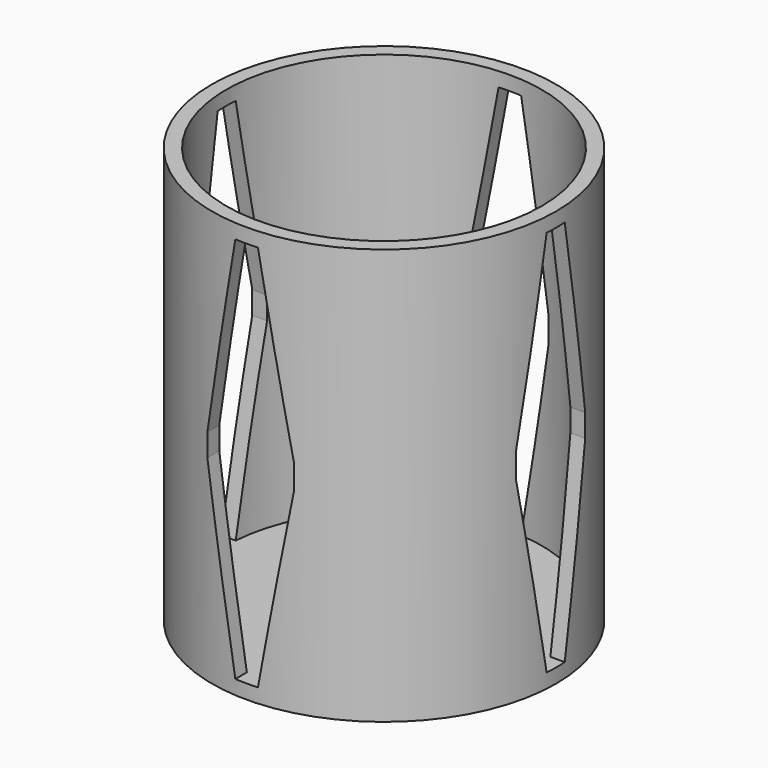
from build123d import *

# Parameters (mm, degrees)
F0_R            = 38.1
F1_DEPTH        = 3.175
F2_R            = 38.1
F2_R_2          = 34.925
F3_DEPTH        = 88.9
F5_DEPTH        = 38.101
F5_COPIES_COUNT = 4


# Not quite as in the source:
# - a pattern or mirror of a feature is missing from the dataset's text; its kind, count and spacing are read off the source's solid


with BuildPart() as f1:
    # F0 (on Top) → F1 (new body)
    with BuildSketch(Plane.XY):
        Circle(F0_R)
    extrude(amount=F1_DEPTH)

    # F2 (on face) → F3 (join)
    with BuildSketch(Plane.XY.offset(3.175)):
        Circle(F2_R)
        Circle(F2_R_2, mode=Mode.SUBTRACT)
    extrude(amount=F3_DEPTH)

    # F4 (on Front) → F5 (cut, through all)
    with BuildSketch(Plane.XZ):
        Polygon((2.5, 88.9), (-2.5, 88.9), (-9.6169977588, 48.5375), (-9.6169977588, 43.5375), (-2.5, 3.175), (2.5, 3.175), (9.6169977588, 43.5375), (9.6169977588, 48.5375), align=None)
    f5 = extrude(amount=-F5_DEPTH, mode=Mode.SUBTRACT)

    # F5_copies: F5 ×4 about axis
    f5_copies_axis = Axis((0, 0, 0), (0, 0, 1))
    for i in range(1, F5_COPIES_COUNT):
        add(f5.rotate(f5_copies_axis, i * 360 / F5_COPIES_COUNT), mode=Mode.SUBTRACT)


solid = f1.part
